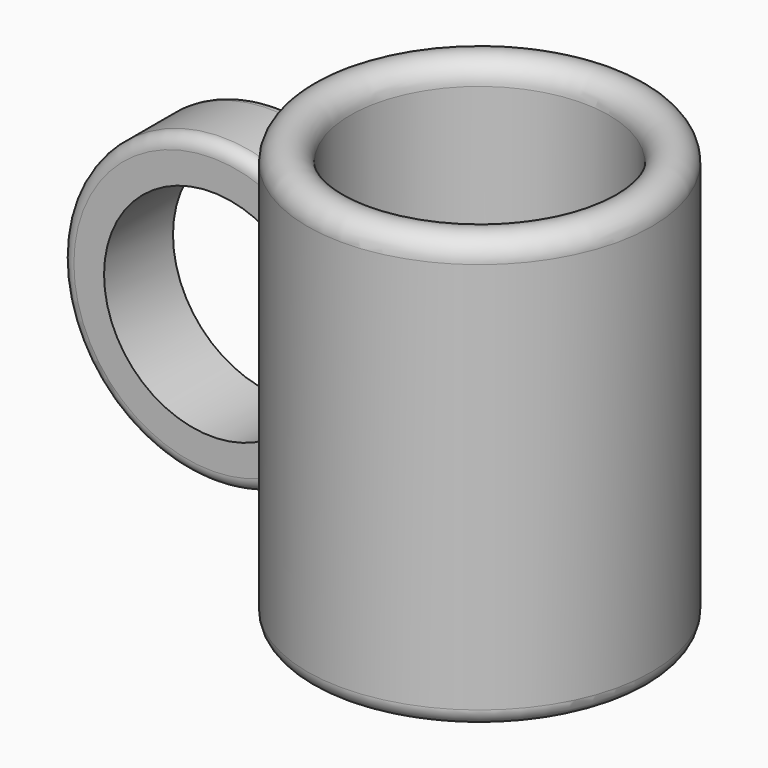
from build123d import *

# Parameters (mm, degrees)
F3_DEPTH = 5
F4_R     = 1.5
F5_R     = 2


# Not quite as in the source:
# - a feature names something its author has since deleted; it is built from what else it names


with BuildPart() as f1:
    # F0 (on Front) → F1 (revolve)
    with BuildSketch(Plane.XZ):
        Polygon((35, 0), (40, 0), (40, 47.5), (35, 47.5), (35, 2.5), align=None)
        with BuildLine():
            Line((35, 47.5), (40, 47.5))
            ThreePointArc((40, 47.5), (37.5, 50), (35, 47.5))
        make_face()
        with BuildLine():
            ThreePointArc((20, 2.5), (27.6034531629, 1.8707189772), (35, 0))
            Line((35, 0), (35, 2.5))
            ThreePointArc((35, 2.5), (27.6034531629, 4.3707189772), (20, 5))
            Line((20, 5), (20, 2.5))
        make_face()
    revolve(axis=Axis((20, 0, 1.25), (0, 0, 1)))

    # F2 (on Front) → F3 (join, symmetric)
    with BuildSketch(Plane.XZ):
        with BuildLine():
            ThreePointArc((1.5, 16.1636090773), (-19.5841423567, 25.25), (1.5, 34.3363909227))
            Line((1.5, 34.3363909227), (1.5, 40.5))
            ThreePointArc((1.5, 40.5), (-24.5841423567, 25.25), (1.5, 10))
            Line((1.5, 10), (1.5, 16.1636090773))
        make_face()
    extrude(amount=F3_DEPTH, both=True)

    # F4
    f4_edges = [f1.edges().sort_by_distance(p)[0] for p in [
        (-24.584142, 5, 25.25),
        (-24.584142, -5, 25.25),
    ]]
    fillet(f4_edges, radius=F4_R)

    # F5
    f5_edges = [f1.edges().sort_by_distance(p)[0] for p in [
        (0, 0, 0),
    ]]
    fillet(f5_edges, radius=F5_R)


solid = f1.part
